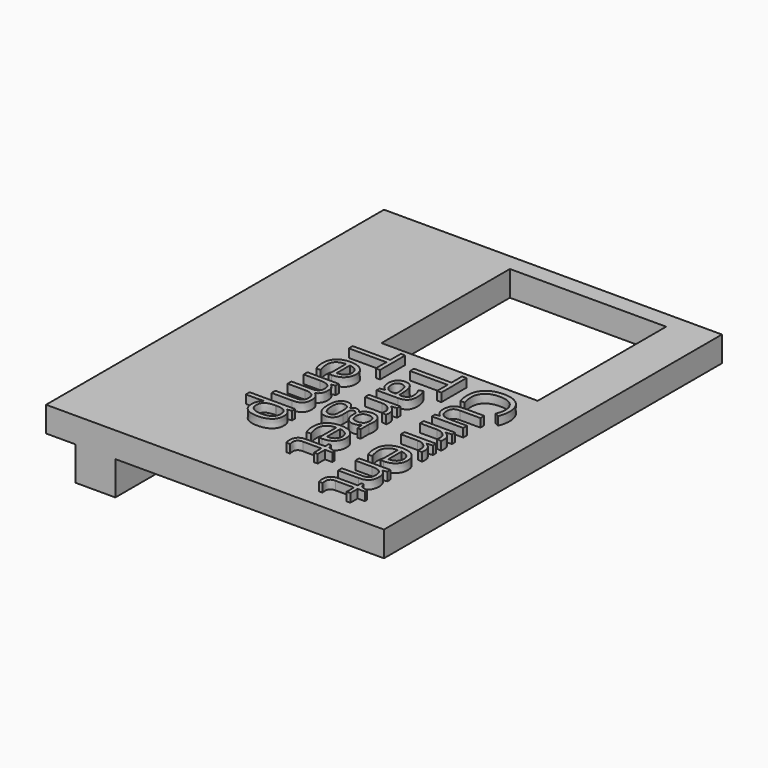
from build123d import *

# Parameters (mm, degrees)
F0_W         = 31.8
F0_H         = 50
F0_W_2       = 18.5
F0_H_2       = 19
F0_W_3       = 1.7
F0_H_3       = 2.5
F0_W_4       = 3.5
F0_H_4       = 45
F1_DEPTH     = 3
F2_DEPTH     = 4
F3_TEXT_SIZE = 6.9444444444
F4_DEPTH     = 1


# Not quite as in the source:
# - a feature names something its author has since deleted; it is built from what else it names
# - Text() gives the source's letters only with a copy of the font that has no kerning and outlines rounded to 1/6400 em; it was checked with that copy


with BuildPart() as f1:
    # F0 (on Top) → F1 (new body)
    with BuildSketch(Plane.XY):
        with Locations((4.1, 0)):
            Rectangle(F0_W, F0_H)
        with Locations((5.75, 13.5)):
            Rectangle(F0_W_2, F0_H_2, mode=Mode.SUBTRACT)
        Polygon((-11.8, -25), (-11.8, 25), (-13.3, 25), (-13.3, 22.5), (-13.3, -22.5), (-13.3, -25), align=None)
        with Locations((-14.15, 23.75)):
            Rectangle(F0_W_3, F0_H_3)
        Polygon((-15, 22.5), (-15, 25), (-16.5, 25), (-16.5, -25), (-15, -25), (-15, -22.5), align=None)
        with Locations((-14.15, -23.75)):
            Rectangle(F0_W_3, F0_H_3)
        with Locations((-18.25, 0)):
            Rectangle(F0_W_4, F0_H)
        with Locations((-14.15, 0)):
            Rectangle(F0_W_3, F0_H_4)
    extrude(amount=F1_DEPTH)

    # F0 (on Top) → F2 (join)
    with BuildSketch(Plane.XY):
        Polygon((-11.8, -25), (-11.8, 25), (-13.3, 25), (-13.3, 22.5), (-13.3, -22.5), (-13.3, -25), align=None)
        Polygon((-15, 22.5), (-15, 25), (-16.5, 25), (-16.5, -25), (-15, -25), (-15, -22.5), align=None)
        with Locations((-14.15, 23.75)):
            Rectangle(F0_W_3, F0_H_3)
        with Locations((-14.15, -23.75)):
            Rectangle(F0_W_3, F0_H_3)
    extrude(amount=-F2_DEPTH)

    # F3 (on face) → F4 (join)
    with BuildSketch(Plane.XY.offset(3)):
        with Locations(Location((10.5, 2), (0, 0, -90))):
            Text('Current', F3_TEXT_SIZE, font='Open Sans', text_align=(TextAlign.LEFT, TextAlign.BOTTOM))
        with Locations(Location((3.25, 2), (0, 0, -90))):
            Text('Target', F3_TEXT_SIZE, font='Open Sans', text_align=(TextAlign.LEFT, TextAlign.BOTTOM))
        with Locations(Location((-4, 2), (0, 0, -90))):
            Text('Temp', F3_TEXT_SIZE, font='Open Sans', text_align=(TextAlign.LEFT, TextAlign.BOTTOM))
    extrude(amount=F4_DEPTH)


solid = f1.part
